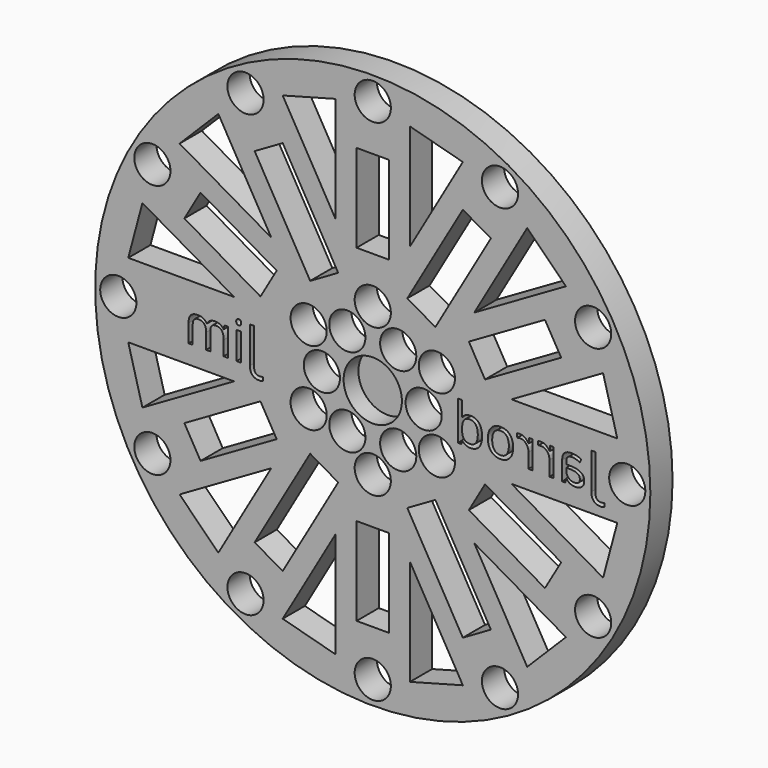
from build123d import *

# Parameters (mm, degrees)
F0_R         = 76.2
F0_R_2       = 4.9657
F0_W         = 8.89
F0_H         = 24.13
F0_R_3       = 8.001
F1_DEPTH     = 7.62
F2_R         = 76.2
F2_R_2       = 4.9657
F2_W         = 8.89
F2_H         = 24.13
F2_R_3       = 8.001
F3_DEPTH     = 2.54
F4_TEXT_SIZE = 14.1111111111
F5_DEPTH     = 7.621
F7_DEPTH     = 7.6210001


# Not quite as in the source:
# - Text() gives the source's letters only with a copy of the font that has no kerning and outlines rounded to 1/6400 em; it was checked with that copy


with BuildPart() as f1:
    # F0 (on Front) → F1 (new body)
    with BuildSketch(Plane.XZ):
        Circle(F0_R)
        with Locations((-34.925, -60.4918744543)):
            Circle(F0_R_2, mode=Mode.SUBTRACT)
        with Locations((-60.4918744543, -34.925)):
            Circle(F0_R_2, mode=Mode.SUBTRACT)
        Polygon((-30.818658833, -12.6605170802), (-26.373658833, -20.3594829198), (-47.2708518263, -32.4244829198), (-51.7158518263, -24.7255170802), align=None, mode=Mode.SUBTRACT)
        Polygon((-9.4855170802, -25.3193975189), (-24.7255170802, -51.7158518263), (-32.4244829198, -47.2708518263), (-17.1844829198, -20.8743975189), align=None, mode=Mode.SUBTRACT)
        with Locations((-17.5976362049, -10.16)):
            Circle(F0_R_2, mode=Mode.SUBTRACT)
        with Locations((-6.985, -12.0983748909)):
            Circle(F0_R_2, mode=Mode.SUBTRACT)
        with Locations((0, -69.85)):
            Circle(F0_R_2, mode=Mode.SUBTRACT)
        with Locations((34.925, -60.4918744543)):
            Circle(F0_R_2, mode=Mode.SUBTRACT)
        with Locations((0, -45.085)):
            Rectangle(F0_W, F0_H, mode=Mode.SUBTRACT)
        with Locations((0, -20.32)):
            Circle(F0_R_2, mode=Mode.SUBTRACT)
        Polygon((17.1844829198, -20.8743975189), (32.4244829198, -47.2708518263), (24.7255170802, -51.7158518263), (9.4855170802, -25.3193975189), align=None, mode=Mode.SUBTRACT)
        with Locations((6.985, -12.0983748909)):
            Circle(F0_R_2, mode=Mode.SUBTRACT)
        with Locations((17.5976362049, -10.16)):
            Circle(F0_R_2, mode=Mode.SUBTRACT)
        Polygon((26.373658833, -20.3594829198), (30.818658833, -12.6605170802), (51.7158518263, -24.7255170802), (47.2708518263, -32.4244829198), align=None, mode=Mode.SUBTRACT)
        with Locations((60.4918744543, -34.925)):
            Circle(F0_R_2, mode=Mode.SUBTRACT)
        with Locations((-69.85, 0)):
            Circle(F0_R_2, mode=Mode.SUBTRACT)
        with Locations((-60.4918744543, 34.925)):
            Circle(F0_R_2, mode=Mode.SUBTRACT)
        Polygon((-26.373658833, 20.3594829198), (-30.818658833, 12.6605170802), (-51.7158518263, 24.7255170802), (-47.2708518263, 32.4244829198), align=None, mode=Mode.SUBTRACT)
        with Locations((-13.97, 0)):
            Circle(F0_R_2, mode=Mode.SUBTRACT)
        with Locations((-17.5976362049, 10.16)):
            Circle(F0_R_2, mode=Mode.SUBTRACT)
        with Locations((-6.985, 12.0983748909)):
            Circle(F0_R_2, mode=Mode.SUBTRACT)
        Polygon((-17.1844829198, 20.8743975189), (-32.4244829198, 47.2708518263), (-24.7255170802, 51.7158518263), (-9.4855170802, 25.3193975189), align=None, mode=Mode.SUBTRACT)
        with Locations((-34.925, 60.4918744543)):
            Circle(F0_R_2, mode=Mode.SUBTRACT)
        Circle(F0_R_3, mode=Mode.SUBTRACT)
        with Locations((13.97, 0)):
            Circle(F0_R_2, mode=Mode.SUBTRACT)
        with Locations((6.985, 12.0983748909)):
            Circle(F0_R_2, mode=Mode.SUBTRACT)
        with Locations((17.5976362049, 10.16)):
            Circle(F0_R_2, mode=Mode.SUBTRACT)
        with Locations((0, 20.32)):
            Circle(F0_R_2, mode=Mode.SUBTRACT)
        Polygon((9.4855170802, 25.3193975189), (24.7255170802, 51.7158518263), (32.4244829198, 47.2708518263), (17.1844829198, 20.8743975189), align=None, mode=Mode.SUBTRACT)
        with Locations((69.85, 0)):
            Circle(F0_R_2, mode=Mode.SUBTRACT)
        Polygon((30.818658833, 12.6605170802), (26.373658833, 20.3594829198), (47.2708518263, 32.4244829198), (51.7158518263, 24.7255170802), align=None, mode=Mode.SUBTRACT)
        with Locations((60.4918744543, 34.925)):
            Circle(F0_R_2, mode=Mode.SUBTRACT)
        with Locations((0, 45.085)):
            Rectangle(F0_W, F0_H, mode=Mode.SUBTRACT)
        with Locations((0, 69.85)):
            Circle(F0_R_2, mode=Mode.SUBTRACT)
        with Locations((34.925, 60.4918744543)):
            Circle(F0_R_2, mode=Mode.SUBTRACT)
    extrude(amount=F1_DEPTH)

    # F2 (on face) → F3 (join)
    with BuildSketch(Plane(origin=(0, 0, 0), x_dir=(-1, 0, 0), z_dir=(0, 1, 0))):
        Circle(F2_R)
        with Locations((-34.925, -60.4918744543)):
            Circle(F2_R_2, mode=Mode.SUBTRACT)
        with Locations((-60.4918744543, -34.925)):
            Circle(F2_R_2, mode=Mode.SUBTRACT)
        Polygon((-51.7158518263, -24.7255170802), (-30.818658833, -12.6605170802), (-26.373658833, -20.3594829198), (-47.2708518263, -32.4244829198), align=None, mode=Mode.SUBTRACT)
        Polygon((-32.4244829198, -47.2708518263), (-17.1844829198, -20.8743975189), (-9.4855170802, -25.3193975189), (-24.7255170802, -51.7158518263), align=None, mode=Mode.SUBTRACT)
        with Locations((-17.5976362049, -10.16)):
            Circle(F2_R_2, mode=Mode.SUBTRACT)
        with Locations((-6.985, -12.0983748909)):
            Circle(F2_R_2, mode=Mode.SUBTRACT)
        with Locations((0, -69.85)):
            Circle(F2_R_2, mode=Mode.SUBTRACT)
        with Locations((34.925, -60.4918744543)):
            Circle(F2_R_2, mode=Mode.SUBTRACT)
        with Locations((0, -45.085)):
            Rectangle(F2_W, F2_H, mode=Mode.SUBTRACT)
        with Locations((0, -20.32)):
            Circle(F2_R_2, mode=Mode.SUBTRACT)
        Polygon((32.4244829198, -47.2708518263), (24.7255170802, -51.7158518263), (9.4855170802, -25.3193975189), (17.1844829198, -20.8743975189), align=None, mode=Mode.SUBTRACT)
        with Locations((6.985, -12.0983748909)):
            Circle(F2_R_2, mode=Mode.SUBTRACT)
        with Locations((17.5976362049, -10.16)):
            Circle(F2_R_2, mode=Mode.SUBTRACT)
        Polygon((30.818658833, -12.6605170802), (51.7158518263, -24.7255170802), (47.2708518263, -32.4244829198), (26.373658833, -20.3594829198), align=None, mode=Mode.SUBTRACT)
        with Locations((60.4918744543, -34.925)):
            Circle(F2_R_2, mode=Mode.SUBTRACT)
        with Locations((-69.85, 0)):
            Circle(F2_R_2, mode=Mode.SUBTRACT)
        with Locations((-60.4918744543, 34.925)):
            Circle(F2_R_2, mode=Mode.SUBTRACT)
        Polygon((-47.2708518263, 32.4244829198), (-26.373658833, 20.3594829198), (-30.818658833, 12.6605170802), (-51.7158518263, 24.7255170802), align=None, mode=Mode.SUBTRACT)
        with Locations((-13.97, 0)):
            Circle(F2_R_2, mode=Mode.SUBTRACT)
        with Locations((-17.5976362049, 10.16)):
            Circle(F2_R_2, mode=Mode.SUBTRACT)
        with Locations((-6.985, 12.0983748909)):
            Circle(F2_R_2, mode=Mode.SUBTRACT)
        Polygon((-9.4855170802, 25.3193975189), (-17.1844829198, 20.8743975189), (-32.4244829198, 47.2708518263), (-24.7255170802, 51.7158518263), align=None, mode=Mode.SUBTRACT)
        with Locations((-34.925, 60.4918744543)):
            Circle(F2_R_2, mode=Mode.SUBTRACT)
        Circle(F2_R_3, mode=Mode.SUBTRACT)
        with Locations((13.97, 0)):
            Circle(F2_R_2, mode=Mode.SUBTRACT)
        with Locations((6.985, 12.0983748909)):
            Circle(F2_R_2, mode=Mode.SUBTRACT)
        with Locations((17.5976362049, 10.16)):
            Circle(F2_R_2, mode=Mode.SUBTRACT)
        with Locations((0, 20.32)):
            Circle(F2_R_2, mode=Mode.SUBTRACT)
        Polygon((17.1844829198, 20.8743975189), (9.4855170802, 25.3193975189), (24.7255170802, 51.7158518263), (32.4244829198, 47.2708518263), align=None, mode=Mode.SUBTRACT)
        with Locations((69.85, 0)):
            Circle(F2_R_2, mode=Mode.SUBTRACT)
        Polygon((51.7158518263, 24.7255170802), (30.818658833, 12.6605170802), (26.373658833, 20.3594829198), (47.2708518263, 32.4244829198), align=None, mode=Mode.SUBTRACT)
        with Locations((60.4918744543, 34.925)):
            Circle(F2_R_2, mode=Mode.SUBTRACT)
        with Locations((0, 45.085)):
            Rectangle(F2_W, F2_H, mode=Mode.SUBTRACT)
        with Locations((0, 69.85)):
            Circle(F2_R_2, mode=Mode.SUBTRACT)
        with Locations((34.925, 60.4918744543)):
            Circle(F2_R_2, mode=Mode.SUBTRACT)
        Circle(F2_R_3)
    extrude(amount=-F3_DEPTH)

    # F4 (on face) → F5 (cut, through all)
    with BuildSketch(Plane(origin=(0, 0, 0), x_dir=(-1, 0, 0), z_dir=(0, 1, 0))):
        with Locations((-62.4670225694, -5.08)):
            Text('Jarrod', F4_TEXT_SIZE, font='Open Sans', text_align=(TextAlign.LEFT, TextAlign.BOTTOM))
        with Locations((31.2417795139, -5.08)):
            Text('Jim', F4_TEXT_SIZE, font='Open Sans', text_align=(TextAlign.LEFT, TextAlign.BOTTOM))
    extrude(amount=-F5_DEPTH, mode=Mode.SUBTRACT)

    # F6 (on face) → F7 (cut, through all)
    with BuildSketch(Plane(origin=(0, 0, 0), x_dir=(-1, 0, 0), z_dir=(0, 1, 0))):
        Polygon((-42.3915397082, 53.0253347461), (-53.0253347461, 42.3915397082), (-27.8655055479, 27.8655055479), align=None)
        Polygon((-63.2248176659, 24.7255170802), (-67.1170567884, 10.1994829198), (-38.0649884677, 10.1994829198), align=None)
        Polygon((-67.1170567884, -10.1994829198), (-63.2248176659, -24.7255170802), (-38.0649884677, -10.1994829198), align=None)
        Polygon((-53.0253347461, -42.3915397082), (-42.3915397082, -53.0253347461), (-27.8655055479, -27.8655055479), align=None)
        Polygon((-24.7255170802, -63.2248176659), (-10.1994829198, -67.1170567884), (-10.1994829198, -38.0649884677), align=None)
        Polygon((10.1994829198, -67.1170567884), (24.7255170802, -63.2248176659), (10.1994829198, -38.0649884677), align=None)
        Polygon((42.3915397082, -53.0253347461), (53.0253347461, -42.3915397082), (27.8655055479, -27.8655055479), align=None)
        Polygon((63.2248176659, -24.7255170802), (67.1170567884, -10.1994829198), (38.0649884677, -10.1994829198), align=None)
        Polygon((67.1170567884, 10.1994829198), (63.2248176659, 24.7255170802), (38.0649884677, 10.1994829198), align=None)
        Polygon((53.0253347461, 42.3915397082), (42.3915397082, 53.0253347461), (27.8655055479, 27.8655055479), align=None)
        Polygon((10.1994829198, 67.1170567884), (10.1994829198, 38.0649884677), (24.7255170802, 63.2248176659), align=None)
        Polygon((-10.1994829198, 67.1170567884), (-24.7255170802, 63.2248176659), (-10.1994829198, 38.0649884677), align=None)
    extrude(amount=-F7_DEPTH, mode=Mode.SUBTRACT)


solid = f1.part
